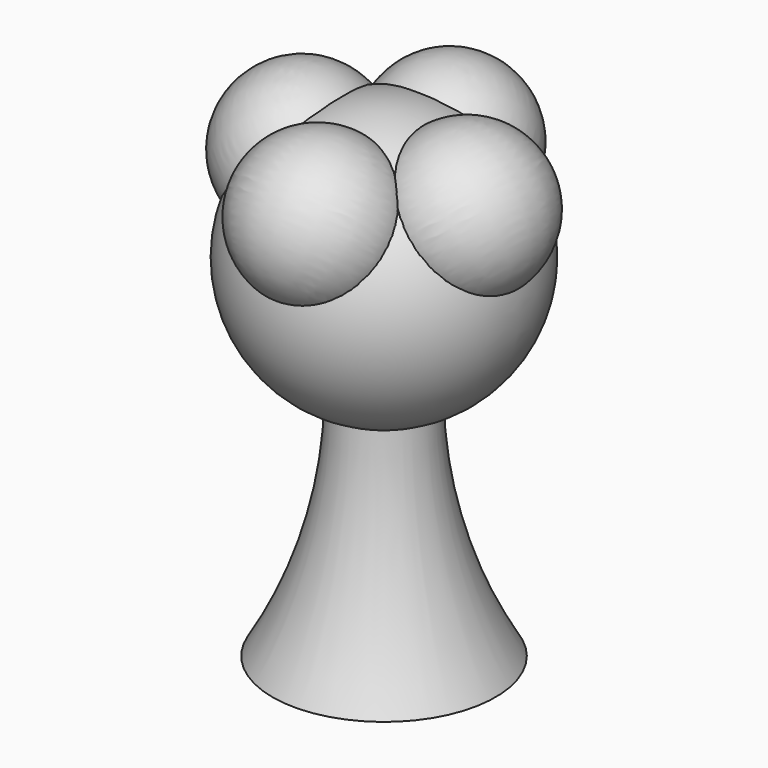
from build123d import *

# Parameters (mm, degrees)
F6_COUNT = 4


with BuildPart() as f1:
    # F0 (on Front) → F1 (revolve)
    with BuildSketch(Plane.XZ):
        with BuildLine():
            ThreePointArc((-22.9558888823, 54.5034594834), (-19.4744061523, -12.9478245932), (-42.2871634364, -76.5196308494))
            Line((-42.2871634364, -76.5196308494), (0, -75.9826526046))
            Line((0, -75.9826526046), (0, 54.5034594834))
            Line((0, 54.5034594834), (-22.9558888823, 54.5034594834))
        make_face()
    revolve(axis=Axis((0, 0, -10.7395965606), (0, 0, -1)))

    # F2 (on Front) → F3 (revolve)
    with BuildSketch(Plane.XZ):
        with BuildLine():
            Line((0, 107.9355524428), (0, 5.2852062933))
            ThreePointArc((0, 5.2852062933), (51.3251730747, 56.6103793681), (0, 107.9355524428))
        make_face()
    revolve(axis=Axis((0, 0, 56.6103793681), (0, 0, 1)))


with BuildPart() as f5:
    # F4 (on Right) → F5 (revolve)
    with BuildSketch(Plane.YZ):
        with BuildLine():
            Line((13.7554751296, 104.4943882979), (48.2909788504, 60.281846064))
            ThreePointArc((48.2909788504, 60.281846064), (53.4677473917, 99.9200838737), (13.7554751296, 104.4943882979))
        make_face()
    revolve(axis=Axis((0, 31.02322699, 82.388117181), (0, 0.6155826648, -0.7880723208)))


with BuildPart() as f6_1:
    # F6: instance of F5
    add(f5.part.rotate(Axis((0, 0, -76.5196308494), (0, 0, -1)), 1 * 360 / F6_COUNT))


with BuildPart() as f6_2:
    # F6: instance of F5
    add(f5.part.rotate(Axis((0, 0, -76.5196308494), (0, 0, -1)), 2 * 360 / F6_COUNT))


with BuildPart() as f6_3:
    # F6: instance of F5
    add(f5.part.rotate(Axis((0, 0, -76.5196308494), (0, 0, -1)), 3 * 360 / F6_COUNT))


solid = Compound([f1.part, f5.part, f6_1.part, f6_2.part, f6_3.part])
